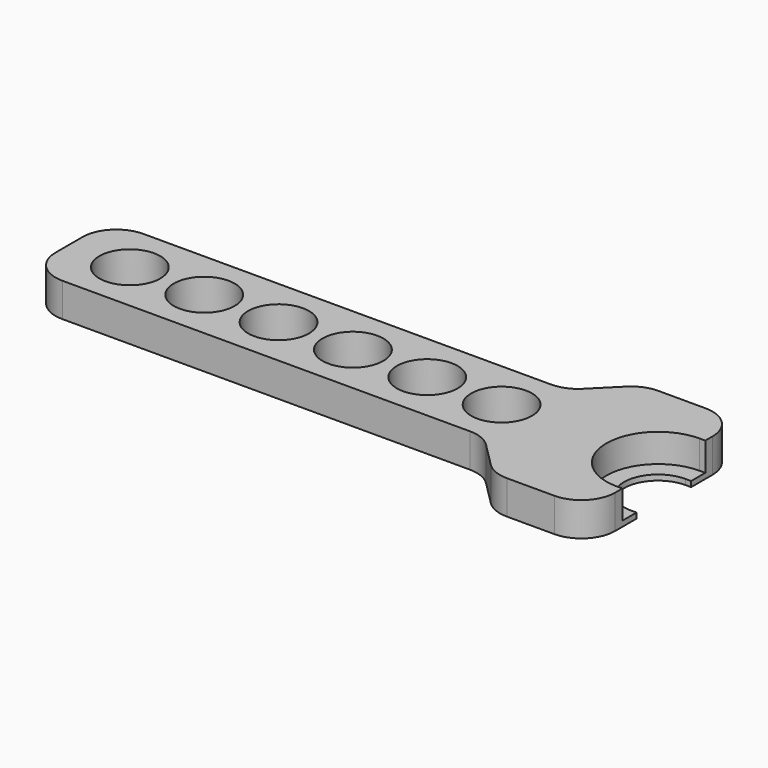
from build123d import *

# Parameters (mm, degrees)
F1_DEPTH    = 6.35
F3_DEPTH    = 5.334
F4_W        = 17.78
F4_H        = 8.255
F5_DEPTH    = 25.4
F6_R        = 5.715
F7_DEPTH    = 25.4
F8_T4_DEPTH = 6.35
F8_T9_DEPTH = 6.35
F9_R        = 6.35


# Not quite as in the source:
# - a fillet or chamfer that OpenCascade refuses, or shapes differently, is made with other operations: its cross-section is extruded or revolved along the edge and cut away or added


with BuildPart() as f1:
    # F0 (on Top) → F1 (new body)
    with BuildSketch(Plane.XY):
        Polygon((8.1444730278, -17.78), (17.78, -17.78), (17.78, 17.78), (-17.78, 17.78), (-17.78, 9.525), (-93.98, 9.525), (-93.98, -9.525), (-17.78, -9.525), (-17.78, -17.78), (-8.1444730278, -17.78), align=None)
    extrude(amount=F1_DEPTH)

    # F2 (on face) → F3 (cut)
    with BuildSketch(Plane.XY.offset(6.35)):
        with BuildLine():
            Line((17.78, 9.7409), (16.7259, 9.7409))
            ThreePointArc((16.7259, 9.7409), (6.985, 0), (16.7259, -9.7409))
            Line((16.7259, -9.7409), (17.78, -9.7409))
            Line((17.78, -9.7409), (17.78, 9.7409))
        make_face()
    extrude(amount=-F3_DEPTH, mode=Mode.SUBTRACT)

    # F4 (on face) → F5 (cut)
    with BuildSketch(Plane(origin=(0, 0, 0), x_dir=(1, 0, 0), z_dir=(0, 0, -1))):
        with BuildLine():
            Line((17.78, 6.4135), (16.7005, 6.4135))
            ThreePointArc((16.7005, 6.4135), (10.287, 0), (16.7005, -6.4135))
            Line((16.7005, -6.4135), (17.78, -6.4135))
            Line((17.78, -6.4135), (17.78, 6.4135))
        make_face()
        with Locations((-8.89, -13.6525)):
            Rectangle(F4_W, F4_H)
        with Locations((-8.89, 13.6525)):
            Rectangle(F4_W, F4_H)
    extrude(amount=-F5_DEPTH, mode=Mode.SUBTRACT)

    # F6 (on face) → F7 (cut)
    with BuildSketch(Plane.XY.offset(6.35)):
        with Locations((-82.55, 0)):
            Circle(F6_R)
        with Locations((-68.58, 0)):
            Circle(F6_R)
        with Locations((-54.61, 0)):
            Circle(F6_R)
        with Locations((-40.64, 0)):
            Circle(F6_R)
        with Locations((-26.67, 0)):
            Circle(F6_R)
        with Locations((-12.7, 0)):
            Circle(F6_R)
    extrude(amount=-F7_DEPTH, mode=Mode.SUBTRACT)

    # F8: chamfer of 8.382 on 2 edges, made by hand


with BuildPart() as f8_tool2:
    # F8_s3 → F8_t4 (new body)
    with BuildSketch(Plane.XY):
        Polygon((0, -17.907), (-8.382, -9.525), (0, -9.525), align=None)
    extrude(amount=F8_T4_DEPTH)

    split(bisect_by=Plane.XZ.offset(17.78), keep=Keep.BOTTOM)


with BuildPart() as f1_1:
    add(f1.part)

    # F8_t1: union F8_tool2
    add(f8_tool2.part)


with BuildPart() as f8_tool7:
    # F8_s8 → F8_t9 (new body)
    with BuildSketch(Plane.XY):
        Polygon((-8.382, 9.525), (0, 17.907), (0, 9.525), align=None)
    extrude(amount=F8_T9_DEPTH)

    split(bisect_by=Plane.XZ.offset(-17.78), keep=Keep.TOP)


with BuildPart() as f1_2:
    add(f1_1.part)

    # F8_t6: union F8_tool7
    add(f8_tool7.part)

    # F9
    f9_edges = [f1_2.edges().sort_by_distance(p)[0] for p in [
        (-8.382, -9.525, 3.175),
        (-8.382, 9.525, 3.175),
        (-0.127, 17.78, 3.175),
        (-0.127, -17.78, 3.175),
        (-93.98, 9.525, 3.175),
        (-93.98, -9.525, 3.175),
        (17.78, 17.78, 3.175),
        (17.78, -17.78, 3.175),
    ]]
    fillet(f9_edges, radius=F9_R)


solid = f1_2.part
